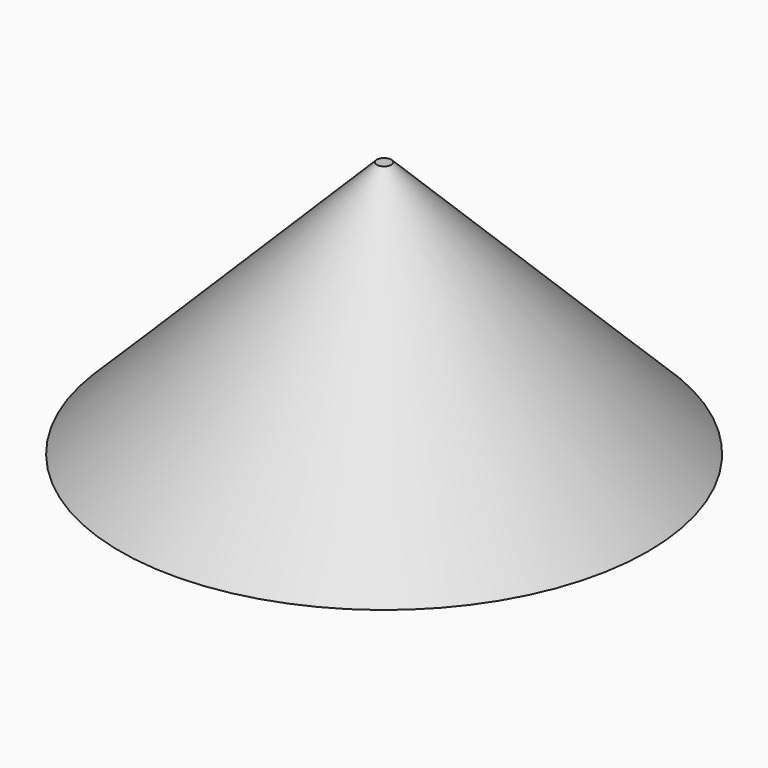
from build123d import *

# Parameters (mm, degrees)
F0_R     = 26.1088044018
F1_DEPTH = 25.4
F1_TAPER = 45


# Not quite as in the source:
# - a feature of the source that left no trace in its solid (it failed there, or was rolled back) is left out


with BuildPart() as f1:
    # F0 (on Top) → F1 (new body)
    with BuildSketch(Plane.XY):
        Circle(F0_R)
    extrude(amount=F1_DEPTH, taper=F1_TAPER)


solid = f1.part
